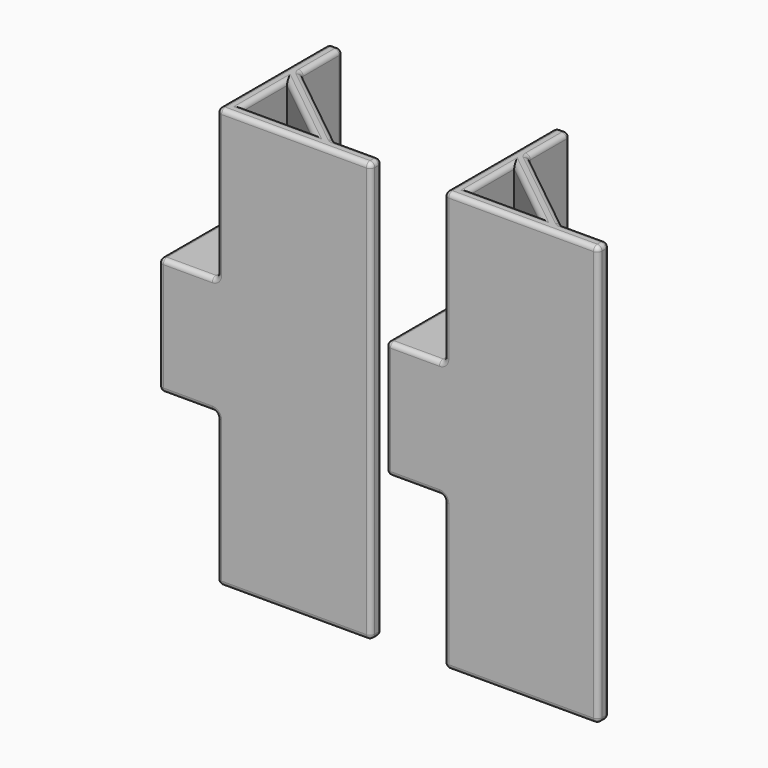
from build123d import *

# Parameters (mm, degrees)
F1_DEPTH = 90
F2_W     = 9.5
F2_H     = 19.25
F3_DEPTH = 3
F4_DEPTH = 30
F6_R     = 1


with BuildPart() as f1:
    # F0 (on Top) → F1 (new body)
    with BuildSketch(Plane.XY):
        Polygon((1.5, 15), (-1.5, 15), (-1.5, -15), (1.5, -15), (1.5, -12), (1.5, 0), (1.5, 3.8418745425), align=None)
        Polygon((21.3023431781, -12), (1.5, 3.8418745425), (1.5, 0), (16.5, -12), align=None)
        Polygon((1.5, -12), (1.5, -15), (31.5, -15), (31.5, -12), (21.3023431781, -12), (16.5, -12), align=None)
    extrude(amount=F1_DEPTH)

    # F2 (on face) → F3 (join)
    with BuildSketch(Plane.XZ.offset(15)):
        with Locations((-6.25, 45)):
            Rectangle(F2_W, F2_H)
    extrude(amount=-F3_DEPTH)

    # F2 (on face) → F4 (join)
    with BuildSketch(Plane.XZ.offset(15)):
        Polygon((-11, 54.625), (-1.5, 54.625), (-1.5, 57.6249994338), (-13.9999994338, 57.6249994338), (-13.9999994338, 32.3750005662), (-1.5, 32.3750005662), (-1.5, 35.375), (-11, 35.375), align=None)
    extrude(amount=-F4_DEPTH)

    # F5: union 

    # F6
    f6_edges = [f1.edges().sort_by_distance(p)[0] for p in [
        (31.5, -12, 45),
        (21.302343, -12, 45),
        (26.401172, -12, 0),
        (26.401172, -12, 90),
        (1.5, 3.841875, 45),
        (11.401172, -4.079063, 0),
        (11.401172, -4.079063, 90),
        (1.5, 15, 45),
        (1.5, 9.420937, 0),
        (1.5, 9.420937, 90),
        (-1.5, 0, 57.624999),
        (-1.5, -15, 73.8125),
        (-1.5, 0, 90),
        (-1.5, 15, 73.8125),
        (-13.999999, 0, 57.624999),
        (-13.999999, 0, 32.375001),
        (-13.999999, -15, 45),
        (-13.999999, 15, 45),
        (-1.5, 0, 0),
        (-1.5, -15, 16.1875),
        (-1.5, 0, 32.375001),
        (-1.5, 15, 16.1875),
        (-7.75, -15, 32.375001),
        (-7.75, -15, 57.624999),
        (15, -15, 90),
        (31.5, -15, 45),
        (15, -15, 0),
        (1.5, -6, 0),
        (9, -6, 0),
        (9, -12, 0),
        (1.5, -6, 90),
        (9, -6, 90),
        (9, -12, 90),
        (0, 15, 90),
        (31.5, -13.5, 90),
        (0, 15, 0),
        (31.5, -13.5, 0),
        (-11, 15, 45),
        (-6.25, 15, 35.375),
        (-1.5, 15, 45),
        (-6.25, 15, 54.625),
        (-7.75, 15, 57.624999),
        (-7.75, 15, 32.375001),
    ]]
    fillet(f6_edges, radius=F6_R)


with BuildPart() as f7_1:
    # F7: copy of F1
    add(f1.part.moved(Location((-48.6, -0.1, 0))))


solid = Compound([f1.part, f7_1.part])
